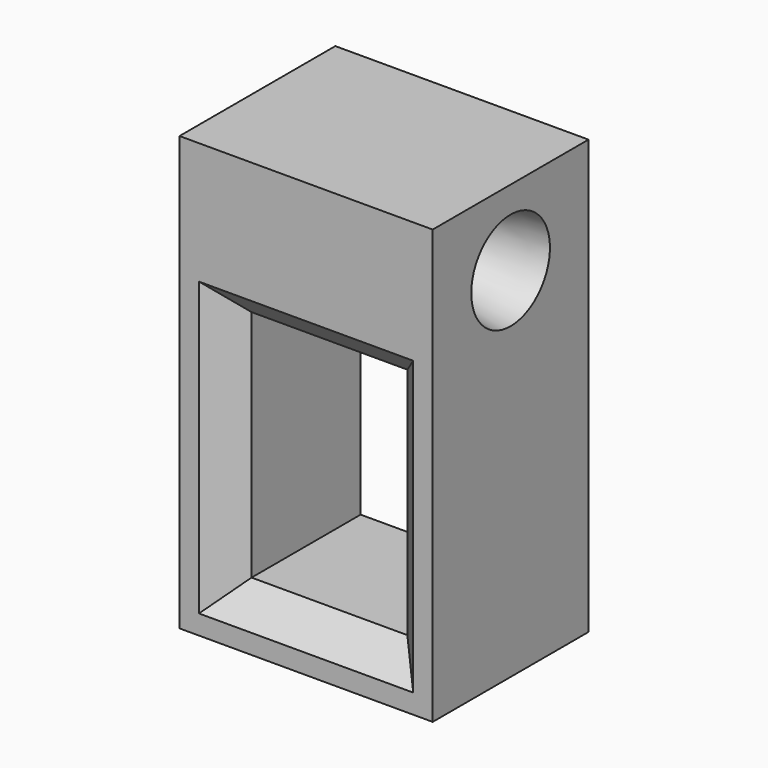
from build123d import *

# Parameters (mm, degrees)
F0_W     = 16.51
F0_H     = 28.265
F0_W_2   = 10.16
F0_H_2   = 15.24
F1_DEPTH = 6.35
F2_SIZE  = 1.905
F4_R     = 1.75
F5_DEPTH = 12.7
F5_TAPER = -10
F6_R     = 12.7


with BuildPart() as f1:
    # F0 (on Front) → F1 (new body, symmetric)
    with BuildSketch(Plane.XZ):
        with Locations((8.255, 14.1325)):
            Rectangle(F0_W, F0_H)
        with Locations((8.255, 10.795)):
            Rectangle(F0_W_2, F0_H_2, mode=Mode.SUBTRACT)
    extrude(amount=F1_DEPTH, both=True)

    # F2
    f2_edges = [f1.edges().sort_by_distance(p)[0] for p in [
        (13.335, -6.35, 10.795),
        (8.255, -6.35, 18.415),
        (3.175, -6.35, 10.795),
        (8.255, -6.35, 3.175),
        (3.175, 6.35, 10.795),
        (8.255, 6.35, 18.415),
        (8.255, 6.35, 3.175),
        (13.335, 6.35, 10.795),
    ]]
    chamfer(f2_edges, length=F2_SIZE)

    # F4 (on mid) → F5 (cut, symmetric)
    with BuildSketch(Plane(origin=(8.255, 0, 0), x_dir=(0, -1, 0), z_dir=(-1, 0, 0))):
        with Locations((0, 23.34)):
            Circle(F4_R)
    extrude(amount=F5_DEPTH, both=True, taper=F5_TAPER, mode=Mode.SUBTRACT)

    # F6
    f6_edges = [f1.edges().sort_by_distance(p)[0] for p in [
        (8.255, 1.75, 23.34),
    ]]
    fillet(f6_edges, radius=F6_R)


solid = f1.part
